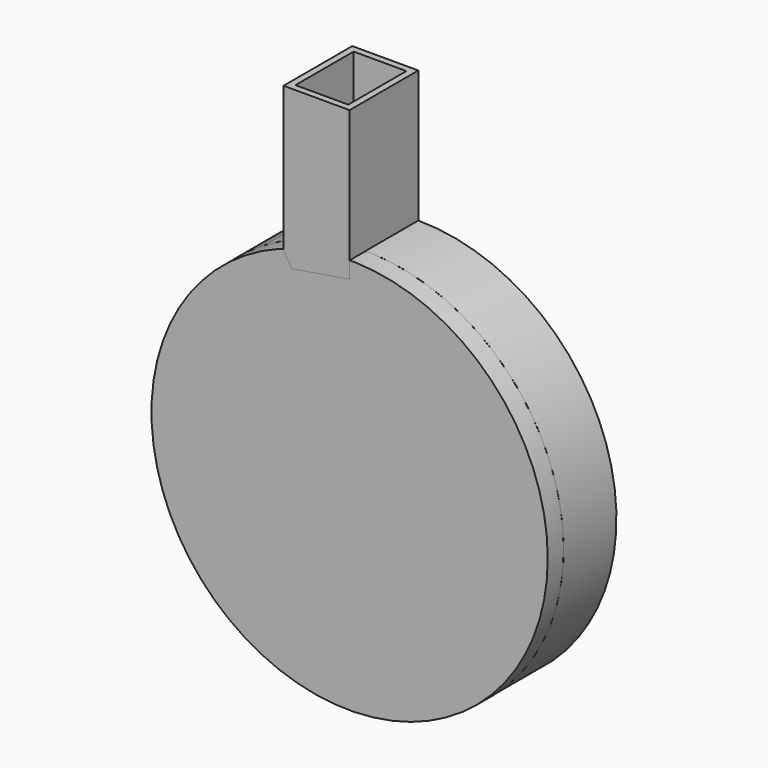
from build123d import *

# Parameters (mm, degrees)
F1_DEPTH      = 12.7
F2_R          = 38.1
F3_DEPTH      = 3.81
F4_T2_ANGLE   = 359.64
F6_DEPTH      = 3.81
F6_DEPTH_BACK = 12.7
F7_T          = -1.27


# Not quite as in the source:
# - a fillet or chamfer that OpenCascade refuses, or shapes differently, is made with other operations: its cross-section is extruded or revolved along the edge and cut away or added


with BuildPart() as f1:
    # F0 (on Front) → F1 (new body)
    with BuildSketch(Plane.XZ):
        with BuildLine():
            ThreePointArc((-8.0861902234, 24.0784868227), (-14.8285327717, -20.6221874649), (25.4, 0))
            ThreePointArc((25.4, 0), (18.5819114233, 17.3168290358), (1.787986783, 25.3369908092))
            ThreePointArc((1.787986783, 25.3369908092), (-3.2113548099, 25.1961743184), (-8.0861902234, 24.0784868227))
        make_face()
    extrude(amount=-F1_DEPTH)


with BuildPart() as f1b:
    # F0 (on Front) → F1, piece 2 (new body)
    with BuildSketch(Plane.XZ):
        with BuildLine():
            Line((0, 38.1), (0.4451874458, 34.9221624923))
            ThreePointArc((0.4451874458, 34.9221624923), (5.4132089756, -34.5029389123), (-11.1185115572, 33.1079193812))
            Line((-11.1185115572, 33.1079193812), (-12.1292853351, 36.1177302341))
            ThreePointArc((-12.1292853351, 36.1177302341), (-12.8456964833, 35.8691801113), (-13.5570191026, 35.6064212334))
            add(Edge.make_bspline(
                [(-13.5570191026, 35.6064212334), (-15.4655091495, 34.6910286845), (-17.3739991965, 33.7756361356), (-19.2824892434, 32.8602435867)],
                knots=[0, 0, 0, 0, 6.35, 6.35, 6.35, 6.35], degree=3))
            ThreePointArc((-19.2824892434, 32.8602435867), (9.9908638101, -36.7667327938), (0, 38.1))
        make_face()
    extrude(amount=-F1_DEPTH)

    # F4: fillet of radius 26.9812507731 on 1 edges, made by hand

    # F4_s1 → F4_t2 (revolve, cut)
    with BuildSketch(Plane(origin=(0, 0, 0), x_dir=(0, 1, 0), z_dir=(-0.9883972718, 0, -0.1518908593))):
        with BuildLine():
            ThreePointArc((12.6984375972, -34.925), (6.1537652905, -35.7307821492), (0, -38.1))
            Line((0, -38.1), (-0.2539687519, -37.6238749845))
            ThreePointArc((-0.2539687519, -37.6238749845), (-0.5396250155, -36.5125), (-0.5396250155, -34.925))
            Line((-0.5396250155, -34.925), (0, -34.3853749845))
            Line((0, -34.3853749845), (12.6984375972, -34.3853749845))
            Line((12.6984375972, -34.3853749845), (12.6984375972, -34.925))
        make_face()
    revolve(axis=Axis((0, 0, 0), (0, 1, 0)), revolution_arc=F4_T2_ANGLE, mode=Mode.SUBTRACT)


with BuildPart() as f3:
    # F2 (on Front) → F3 (new body)
    with BuildSketch(Plane.XZ):
        Circle(F2_R)
    extrude(amount=F3_DEPTH)


with BuildPart() as f6:
    # F5 (on Front) → F6 (new body, two sides)
    with BuildSketch(Plane.XZ) as f6_sk:
        Polygon((-12.7, 35.56), (0, 38.1), (0, 63.5), (-12.7, 63.5), align=None)
        Polygon((-11.1233824864, 33.0410040915), (0, 34.8688024059), (0, 38.1), (-12.7, 35.56), align=None)
    extrude(amount=F6_DEPTH)
    extrude(f6_sk.sketch, amount=-F6_DEPTH_BACK)

    # F7
    f7_openings = [f6.faces().sort_by_distance(p)[0] for p in [
        (-6.35, 4.445, 63.5),
        (-5.561691, 4.445, 33.954903),
    ]]
    offset(amount=F7_T, openings=f7_openings)


solid = Compound([f1.part, f1b.part, f3.part, f6.part])
